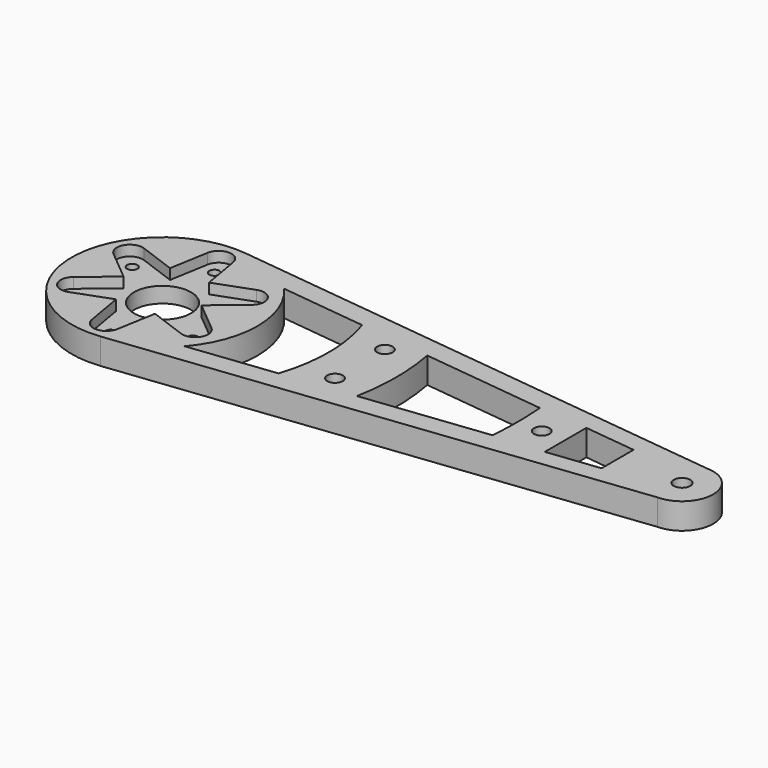
from build123d import *

# Parameters (mm, degrees)
F0_R     = 1.6
F0_R_2   = 5.5
F1_DEPTH = 3
F2_DEPTH = 5
F3_R     = 1
F3_W     = 5
F3_H     = 5
F3_H_2   = 4.5
F3_R_2   = 3.5
F4_DEPTH = 3
F5_R     = 1.5
F6_DEPTH = 25
F7_DEPTH = 25


# Not quite as in the source:
# - a feature names something its author has since deleted; it is built from what else it names


with BuildPart() as f1:
    # F0 (on Top) → F1 (new body)
    with BuildSketch(Plane.XY):
        with BuildLine():
            Line((100.0328712093, 5.9999099563), (2.0188625271, 17.3831583464))
            ThreePointArc((2.0188625271, 17.3831583464), (-17.5, 0), (2.0188625271, -17.3831583464))
            Line((2.0188625271, -17.3831583464), (100.0328712093, -5.9999099563))
            ThreePointArc((100.0328712093, -5.9999099563), (106, 0), (100.0328712093, 5.9999099563))
        make_face()
        with BuildLine():
            ThreePointArc((-2.4633505863, 13.9265019214), (0, 16), (2.4633505863, 13.9265019214))
            Line((2.4633505863, 13.9265019214), (3.75, 6.4951905284))
            Line((3.75, 6.4951905284), (10.8290291566, 9.0965751469))
            ThreePointArc((10.8290291566, 9.0965751469), (13.8564064606, 8), (13.2923797429, 4.8299267745))
            Line((13.2923797429, 4.8299267745), (7.5, 0))
            Line((7.5, 0), (13.2923797429, -4.8299267745))
            ThreePointArc((13.2923797429, -4.8299267745), (13.8564064606, -8), (10.8290291566, -9.0965751469))
            Line((10.8290291566, -9.0965751469), (3.75, -6.4951905284))
            Line((3.75, -6.4951905284), (2.4633505863, -13.9265019214))
            ThreePointArc((2.4633505863, -13.9265019214), (0, -16), (-2.4633505863, -13.9265019214))
            Line((-2.4633505863, -13.9265019214), (-3.75, -6.4951905284))
            Line((-3.75, -6.4951905284), (-10.8290291566, -9.0965751469))
            ThreePointArc((-10.8290291566, -9.0965751469), (-13.8564064606, -8), (-13.2923797429, -4.8299267745))
            Line((-13.2923797429, -4.8299267745), (-7.5, 0))
            Line((-7.5, 0), (-13.2923797429, 4.8299267745))
            ThreePointArc((-13.2923797429, 4.8299267745), (-13.8564064606, 8), (-10.8290291566, 9.0965751469))
            Line((-10.8290291566, 9.0965751469), (-3.75, 6.4951905284))
            Line((-3.75, 6.4951905284), (-2.4633505863, 13.9265019214))
        make_face(mode=Mode.SUBTRACT)
        with BuildLine():
            Line((30.3766267594, -10.0628299558), (13.8329335508, -11.9841978461))
            ThreePointArc((13.8329335508, -11.9841978461), (18.3022143096, 0), (13.8329335508, 11.9841978461))
            Line((13.8329335508, 11.9841978461), (30.3766267594, 10.0628299558))
            ThreePointArc((30.3766267594, 10.0628299558), (32, 0), (30.3766267594, -10.0628299558))
        make_face(mode=Mode.SUBTRACT)
        with BuildLine():
            Line((68.0861847768, -5.6832798143), (44.198061298, -8.4576224495))
            ThreePointArc((44.198061298, -8.4576224495), (45, 0), (44.198061298, 8.4576224495))
            Line((44.198061298, 8.4576224495), (68.0861847768, 5.6832798143))
            ThreePointArc((68.0861847768, 5.6832798143), (68.3229699802, 0), (68.0861847768, -5.6832798143))
        make_face(mode=Mode.SUBTRACT)
        Polygon((77.5869291791, -5), (77.5869291791, 5), (87.5869291791, 3.8386100576), (87.5869291791, -3.8386100576), align=None, mode=Mode.SUBTRACT)
        with Locations((100, 0)):
            Circle(F0_R, mode=Mode.SUBTRACT)
        with BuildLine():
            Line((3.75, 6.4951905284), (2.4633505863, 13.9265019214))
            ThreePointArc((2.4633505863, 13.9265019214), (0, 16), (-2.4633505863, 13.9265019214))
            Line((-2.4633505863, 13.9265019214), (-3.75, 6.4951905284))
            Line((-3.75, 6.4951905284), (-10.8290291566, 9.0965751469))
            ThreePointArc((-10.8290291566, 9.0965751469), (-13.8564064606, 8), (-13.2923797429, 4.8299267745))
            Line((-13.2923797429, 4.8299267745), (-7.5, 0))
            Line((-7.5, 0), (-13.2923797429, -4.8299267745))
            ThreePointArc((-13.2923797429, -4.8299267745), (-13.8564064606, -8), (-10.8290291566, -9.0965751469))
            Line((-10.8290291566, -9.0965751469), (-3.75, -6.4951905284))
            Line((-3.75, -6.4951905284), (-2.4633505863, -13.9265019214))
            ThreePointArc((-2.4633505863, -13.9265019214), (0, -16), (2.4633505863, -13.9265019214))
            Line((2.4633505863, -13.9265019214), (3.75, -6.4951905284))
            Line((3.75, -6.4951905284), (10.8290291566, -9.0965751469))
            ThreePointArc((10.8290291566, -9.0965751469), (13.8564064606, -8), (13.2923797429, -4.8299267745))
            Line((13.2923797429, -4.8299267745), (7.5, 0))
            Line((7.5, 0), (13.2923797429, 4.8299267745))
            ThreePointArc((13.2923797429, 4.8299267745), (13.8564064606, 8), (10.8290291566, 9.0965751469))
            Line((10.8290291566, 9.0965751469), (3.75, 6.4951905284))
        make_face()
        Circle(F0_R_2, mode=Mode.SUBTRACT)
    extrude(amount=F1_DEPTH)

    # F0 (on Top) → F2 (join)
    with BuildSketch(Plane.XY):
        with BuildLine():
            Line((100.0328712093, 5.9999099563), (2.0188625271, 17.3831583464))
            ThreePointArc((2.0188625271, 17.3831583464), (-17.5, 0), (2.0188625271, -17.3831583464))
            Line((2.0188625271, -17.3831583464), (100.0328712093, -5.9999099563))
            ThreePointArc((100.0328712093, -5.9999099563), (106, 0), (100.0328712093, 5.9999099563))
        make_face()
        with BuildLine():
            ThreePointArc((-2.4633505863, 13.9265019214), (0, 16), (2.4633505863, 13.9265019214))
            Line((2.4633505863, 13.9265019214), (3.75, 6.4951905284))
            Line((3.75, 6.4951905284), (10.8290291566, 9.0965751469))
            ThreePointArc((10.8290291566, 9.0965751469), (13.8564064606, 8), (13.2923797429, 4.8299267745))
            Line((13.2923797429, 4.8299267745), (7.5, 0))
            Line((7.5, 0), (13.2923797429, -4.8299267745))
            ThreePointArc((13.2923797429, -4.8299267745), (13.8564064606, -8), (10.8290291566, -9.0965751469))
            Line((10.8290291566, -9.0965751469), (3.75, -6.4951905284))
            Line((3.75, -6.4951905284), (2.4633505863, -13.9265019214))
            ThreePointArc((2.4633505863, -13.9265019214), (0, -16), (-2.4633505863, -13.9265019214))
            Line((-2.4633505863, -13.9265019214), (-3.75, -6.4951905284))
            Line((-3.75, -6.4951905284), (-10.8290291566, -9.0965751469))
            ThreePointArc((-10.8290291566, -9.0965751469), (-13.8564064606, -8), (-13.2923797429, -4.8299267745))
            Line((-13.2923797429, -4.8299267745), (-7.5, 0))
            Line((-7.5, 0), (-13.2923797429, 4.8299267745))
            ThreePointArc((-13.2923797429, 4.8299267745), (-13.8564064606, 8), (-10.8290291566, 9.0965751469))
            Line((-10.8290291566, 9.0965751469), (-3.75, 6.4951905284))
            Line((-3.75, 6.4951905284), (-2.4633505863, 13.9265019214))
        make_face(mode=Mode.SUBTRACT)
        with BuildLine():
            Line((30.3766267594, -10.0628299558), (13.8329335508, -11.9841978461))
            ThreePointArc((13.8329335508, -11.9841978461), (18.3022143096, 0), (13.8329335508, 11.9841978461))
            Line((13.8329335508, 11.9841978461), (30.3766267594, 10.0628299558))
            ThreePointArc((30.3766267594, 10.0628299558), (32, 0), (30.3766267594, -10.0628299558))
        make_face(mode=Mode.SUBTRACT)
        with BuildLine():
            Line((68.0861847768, -5.6832798143), (44.198061298, -8.4576224495))
            ThreePointArc((44.198061298, -8.4576224495), (45, 0), (44.198061298, 8.4576224495))
            Line((44.198061298, 8.4576224495), (68.0861847768, 5.6832798143))
            ThreePointArc((68.0861847768, 5.6832798143), (68.3229699802, 0), (68.0861847768, -5.6832798143))
        make_face(mode=Mode.SUBTRACT)
        Polygon((77.5869291791, -5), (77.5869291791, 5), (87.5869291791, 3.8386100576), (87.5869291791, -3.8386100576), align=None, mode=Mode.SUBTRACT)
        with Locations((100, 0)):
            Circle(F0_R, mode=Mode.SUBTRACT)
    extrude(amount=F2_DEPTH)

    # F3 (on face) → F4 (cut)
    with BuildSketch(Plane.XY):
        with Locations((0, -12.5)):
            Circle(F3_R)
        with Locations((10.8253175473, -6.25)):
            Circle(F3_R)
        with Locations((10.8253175473, 6.25)):
            Circle(F3_R)
        with Locations((0, 12.5)):
            Circle(F3_R)
        with Locations((-10.8253175473, 6.25)):
            Circle(F3_R)
        with Locations((-10.8253175473, -6.25)):
            Circle(F3_R)
        with Locations((38, 6)):
            Rectangle(F3_W, F3_H)
        with Locations((73, 0)):
            Rectangle(F3_W, F3_H_2)
        with Locations((38, -6)):
            Rectangle(F3_W, F3_H)
        with Locations((100.0133901834, 0)):
            Circle(F3_R_2)
    extrude(amount=F4_DEPTH, mode=Mode.SUBTRACT)

    # F5 (on face) → F6 (cut)
    with BuildSketch(Plane.XY):
        with Locations((38, -6)):
            Circle(F5_R)
        with Locations((73, 0)):
            Circle(F5_R)
        with Locations((38, 6)):
            Circle(F5_R)
    extrude(amount=F6_DEPTH, mode=Mode.SUBTRACT)

    # F3 (on face) → F7 (cut)
    with BuildSketch(Plane.XY):
        with Locations((0, -12.5)):
            Circle(F3_R)
        with Locations((10.8253175473, -6.25)):
            Circle(F3_R)
        with Locations((10.8253175473, 6.25)):
            Circle(F3_R)
        with Locations((0, 12.5)):
            Circle(F3_R)
        with Locations((-10.8253175473, 6.25)):
            Circle(F3_R)
        with Locations((-10.8253175473, -6.25)):
            Circle(F3_R)
        with Locations((73, 0)):
            Rectangle(F3_W, F3_H_2)
    extrude(amount=-F7_DEPTH, mode=Mode.SUBTRACT)


solid = f1.part
